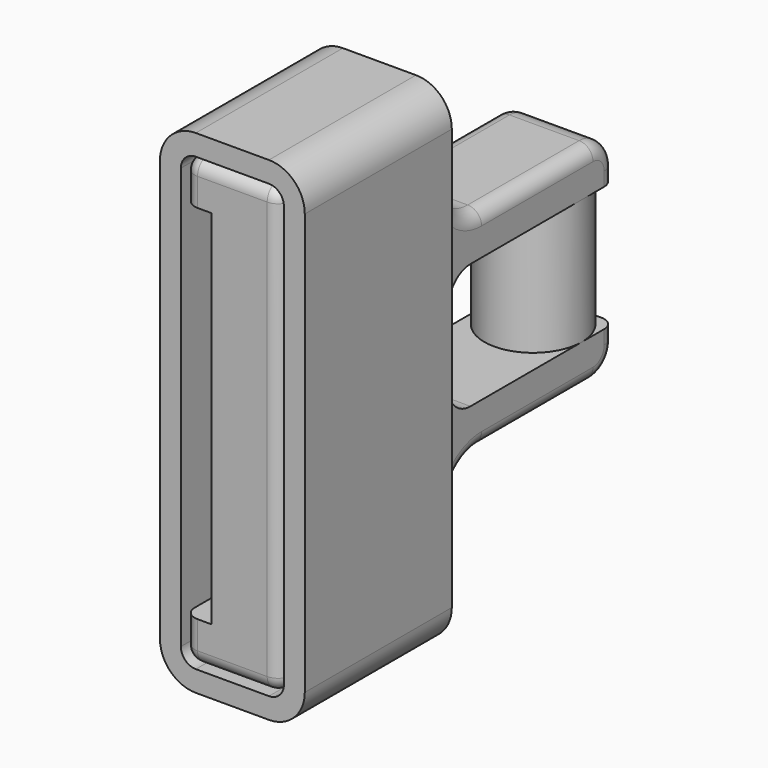
from build123d import *

# Parameters (mm, degrees)
F0_W      = 15
F0_H      = 3
F0_W_2    = 4.5
F0_H_2    = 26
F1_DEPTH  = 3.5
F2_R      = 3.5
F3_DEPTH  = 9
F4_R      = 1
F5_R      = 3
F6_R      = 2
F7_R      = 1
F8_SIZE2  = 3.99999
F8_SIZE   = 6.99999
F9_W      = 4.2
F9_H      = 26
F10_DEPTH = 5
F11_SIZE2 = 3
F11_SIZE  = 4.9
F12_W     = 7.5
F12_H     = 26
F13_DEPTH = 2
F16_DEPTH = 13.2
F17_SIZE  = 1


# Not quite as in the source:
# - a fillet or chamfer is up to 0.001 mm smaller than in the source, because OpenCascade refuses the exact size


with BuildPart() as f1:
    # F0 (on Right) → F1 (new body, symmetric)
    with BuildSketch(Plane.YZ):
        with Locations((-4.5, 6)):
            Rectangle(F0_W, F0_H)
        Polygon((-12, -4.5), (-12, 4.5), (-12, 7.5), (-12, 16), (-27, 16), (-27, -16), (-12, -16), (-12, -7.5), align=None)
        with Locations((-17.25, 0)):
            Rectangle(F0_W_2, F0_H_2, mode=Mode.SUBTRACT)
        with Locations((-4.5, -6)):
            Rectangle(F0_W, F0_H)
    extrude(amount=F1_DEPTH, both=True)

    # F2 (on face) → F3 (join, through all)
    with BuildSketch(Plane.XY.offset(-4.5)):
        Circle(F2_R)
    extrude(amount=F3_DEPTH)

    # F4
    f4_edges = [f1.edges().sort_by_distance(p)[0] for p in [
        (0, -12, 16),
        (0, -12, -16),
        (0, -27, 16),
        (0, -27, -16),
    ]]
    fillet(f4_edges, radius=F4_R)

    # F5
    f5_edges = [f1.edges().sort_by_distance(p)[0] for p in [
        (0, -12, 7.5),
        (0, -12, -7.5),
    ]]
    fillet(f5_edges, radius=F5_R)

    # F6
    f6_edges = [f1.edges().sort_by_distance(p)[0] for p in [
        (0, 3, 7.5),
        (0, 3, -7.5),
        (0, -12, -4.5),
        (0, -12, 4.5),
    ]]
    fillet(f6_edges, radius=F6_R)

    # F7
    f7_edges = [f1.edges().sort_by_distance(p)[0] for p in [
        (3.5, 2.414214, 6.914214),
        (3.5, 2.414214, -6.914214),
        (-3.5, -19.5, -16),
        (-3.5, -19.5, 16),
    ]]
    fillet(f7_edges, radius=F7_R)

    # F8 (size 7 and 4 in the source; OpenCascade refuses exactly that, so slightly less here)
    f8_edges = [f1.edges().sort_by_distance(p)[0] for p in [
        (3.5, -19.5, 0),
    ]]
    f8_side = f1.faces().sort_by_distance((0, -19.5, 0))[0]
    chamfer(f8_edges, length=F8_SIZE, length2=F8_SIZE2, reference=f8_side)

    # F12 (on face) → F13 (cut)
    with BuildSketch(Plane(origin=(-3.5, 0, 0), x_dir=(0, -1, 0), z_dir=(-1, 0, 0))):
        with Locations((23.25, 0)):
            Rectangle(F12_W, F12_H)
    extrude(amount=-F13_DEPTH, mode=Mode.SUBTRACT)


with BuildPart() as f10:
    # F9 (on face) → F10 (new body)
    with BuildSketch(Plane.YZ.offset(3.5)):
        with Locations((-19.1, 0)):
            Rectangle(F9_W, F9_H)
    extrude(amount=-F10_DEPTH)

    # F11
    f11_edges = [f10.edges().sort_by_distance(p)[0] for p in [
        (-1.5, -21.2, 0),
    ]]
    f11_side = f10.faces().sort_by_distance((1, -21.2, 0))[0]
    chamfer(f11_edges, length=F11_SIZE, length2=F11_SIZE2, reference=f11_side)


with BuildPart() as f1_1:
    add(f1.part)

    # F14: union F10
    add(f10.part)


with BuildPart() as f16:
    # F15 (on face) → F16 (new body)
    with BuildSketch(Plane.XZ.offset(27)):
        with BuildLine():
            Line((2.6246717919, 17.7), (-2.6246717919, 17.7))
            ThreePointArc((-2.6246717919, 17.7), (-4.4457038316, 16.9457038316), (-5.2, 15.1246717919))
            Line((-5.2, 15.1246717919), (-5.2, -15.1246717919))
            ThreePointArc((-5.2, -15.1246717919), (-4.4457038316, -16.9457038316), (-2.6246717919, -17.7))
            Line((-2.6246717919, -17.7), (2.6246717919, -17.7))
            ThreePointArc((2.6246717919, -17.7), (4.4457038316, -16.9457038316), (5.2, -15.1246717919))
            Line((5.2, -15.1246717919), (5.2, 15.1246717919))
            ThreePointArc((5.2, 15.1246717919), (4.4457038316, 16.9457038316), (2.6246717919, 17.7))
        make_face()
        with BuildLine():
            Line((-2.6246717919, 16.2), (2.6246717919, 16.2))
            ThreePointArc((2.6246717919, 16.2), (3.3850436598, 15.8850436598), (3.7, 15.1246717919))
            Line((3.7, 15.1246717919), (3.7, -15.1246717919))
            ThreePointArc((3.7, -15.1246717919), (3.3850436598, -15.8850436598), (2.6246717919, -16.2))
            Line((2.6246717919, -16.2), (-2.6246717919, -16.2))
            ThreePointArc((-2.6246717919, -16.2), (-3.3850436598, -15.8850436598), (-3.7, -15.1246717919))
            Line((-3.7, -15.1246717919), (-3.7, 15.1246717919))
            ThreePointArc((-3.7, 15.1246717919), (-3.3850436598, 15.8850436598), (-2.6246717919, 16.2))
        make_face(mode=Mode.SUBTRACT)
    extrude(amount=-F16_DEPTH)

    # F17
    f17_edges = [f16.edges().sort_by_distance(p)[0] for p in [
        (-3.7, -13.8, 0),
    ]]
    chamfer(f17_edges, length=F17_SIZE)


solid = Compound([f1_1.part, f16.part])
